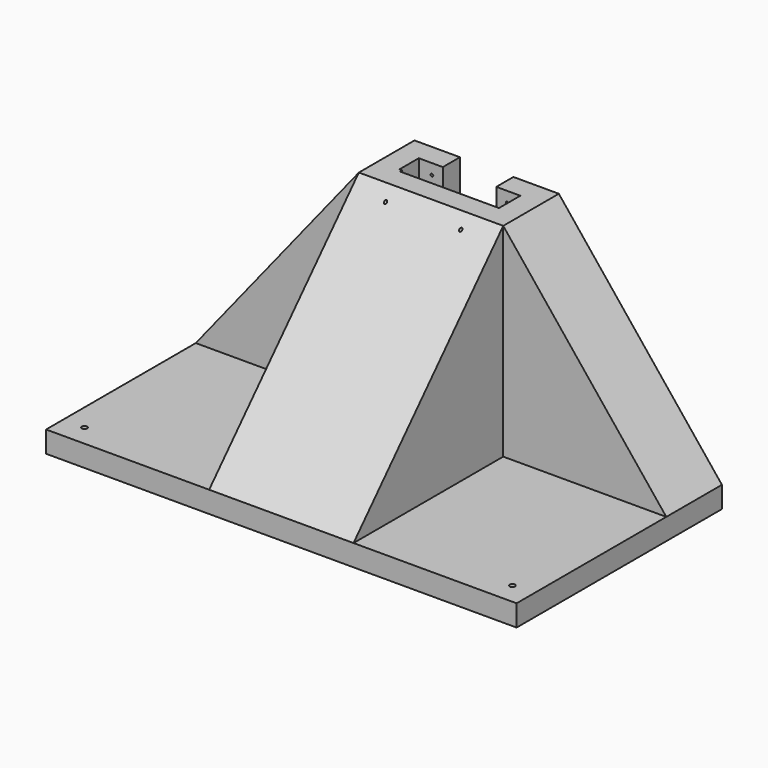
from build123d import *

# Parameters (mm, degrees)
F1_DEPTH  = 533.4
F0_R      = 6.35
F2_DEPTH  = 50.8
F4_DEPTH  = 171.45
F6_DEPTH  = 165.1
F7_R      = 3.175
F8_DEPTH  = 88.9
F9_R      = 3.175
F10_DEPTH = 25.4
F11_R     = 3.175
F12_DEPTH = 25.4
F13_W     = 6.35
F13_H     = 6.35
F14_DEPTH = 533.4


# Not quite as in the source:
# - a feature names something its author has since deleted; it is built from what else it names


with BuildPart() as f1:
    # F0 (on Top) → F1 (new body)
    with BuildSketch(Plane.XY):
        Polygon((-171.45, 165.1), (-171.45, 0), (171.45, 0), (171.45, 165.1), (63.5, 165.1), (63.5, 114.3), (120.65, 114.3), (120.65, 50.8), (-120.65, 50.8), (-120.65, 114.3), (-63.5, 114.3), (-63.5, 165.1), align=None)
    extrude(amount=F1_DEPTH)

    # F0 (on Top) → F2 (join)
    with BuildSketch(Plane.XY):
        Polygon((-171.45, 165.1), (-171.45, 0), (171.45, 0), (171.45, 165.1), (63.5, 165.1), (63.5, 114.3), (120.65, 114.3), (120.65, 50.8), (-120.65, 50.8), (-120.65, 114.3), (-63.5, 114.3), (-63.5, 165.1), align=None)
        Polygon((171.45, 0), (-171.45, 0), (-171.45, 165.1), (-558.8, 165.1), (-558.8, -444.5), (558.8, -444.5), (558.8, 165.1), (171.45, 165.1), align=None)
        with Locations((-508, -393.7)):
            Circle(F0_R, mode=Mode.SUBTRACT)
        with Locations((508, -393.7)):
            Circle(F0_R, mode=Mode.SUBTRACT)
    extrude(amount=F2_DEPTH)

    # F3 (on Right) → F4 (join, symmetric)
    with BuildSketch(Plane.YZ):
        Polygon((-444.5, 50.8), (0, 50.8), (0, 533.4), align=None)
    extrude(amount=F4_DEPTH, both=True)

    # F5 (on face) → F6 (join)
    with BuildSketch(Plane(origin=(0, 165.1, 0), x_dir=(-1, 0, 0), z_dir=(0, 1, 0))):
        Polygon((-558.8, 50.8), (-171.45, 50.8), (-171.45, 533.4), align=None)
        Polygon((171.45, 533.4), (171.45, 50.8), (558.8, 50.8), align=None)
    extrude(amount=-F6_DEPTH)

    # F7 (on face) → F8 (cut, symmetric)
    with BuildSketch(Plane(origin=(0, 50.8, 0), x_dir=(-1, 0, 0), z_dir=(0, 1, 0))):
        with Locations((-89.2969816923, 146.05)):
            Circle(F7_R)
        with Locations((-89.2969816923, 266.7)):
            Circle(F7_R)
        with Locations((-89.2969816923, 25.4)):
            Circle(F7_R)
        with Locations((-89.2969816923, 508)):
            Circle(F7_R)
        with Locations((-89.2969816923, 387.35)):
            Circle(F7_R)
        with Locations((89.2969816923, 25.4)):
            Circle(F7_R)
        with Locations((89.2969816923, 146.05)):
            Circle(F7_R)
        with Locations((89.2969816923, 266.7)):
            Circle(F7_R)
        with Locations((89.2969816923, 387.35)):
            Circle(F7_R)
        with Locations((89.2969816923, 508)):
            Circle(F7_R)
    extrude(amount=F8_DEPTH, both=True, mode=Mode.SUBTRACT)

    # F9 (on face) → F10 (cut)
    with BuildSketch(Plane(origin=(120.65, 0, 0), x_dir=(0, -1, 0), z_dir=(-1, 0, 0))):
        with Locations((-82.55, 25.4)):
            Circle(F9_R)
        with Locations((-82.55, 146.05)):
            Circle(F9_R)
        with Locations((-82.55, 266.7)):
            Circle(F9_R)
        with Locations((-82.55, 387.35)):
            Circle(F9_R)
        with Locations((-82.55, 508)):
            Circle(F9_R)
    extrude(amount=-F10_DEPTH, mode=Mode.SUBTRACT)

    # F11 (on face) → F12 (cut)
    with BuildSketch(Plane.YZ.offset(-120.65)):
        with Locations((82.55, 25.4)):
            Circle(F11_R)
        with Locations((82.55, 146.05)):
            Circle(F11_R)
        with Locations((82.55, 266.7)):
            Circle(F11_R)
        with Locations((82.55, 387.35)):
            Circle(F11_R)
        with Locations((82.55, 508)):
            Circle(F11_R)
    extrude(amount=-F12_DEPTH, mode=Mode.SUBTRACT)

    # F13 (on Top) → F14 (join)
    with BuildSketch(Plane.XY):
        with Locations((-117.475, 53.975)):
            Rectangle(F13_W, F13_H)
    extrude(amount=F14_DEPTH)


solid = f1.part
